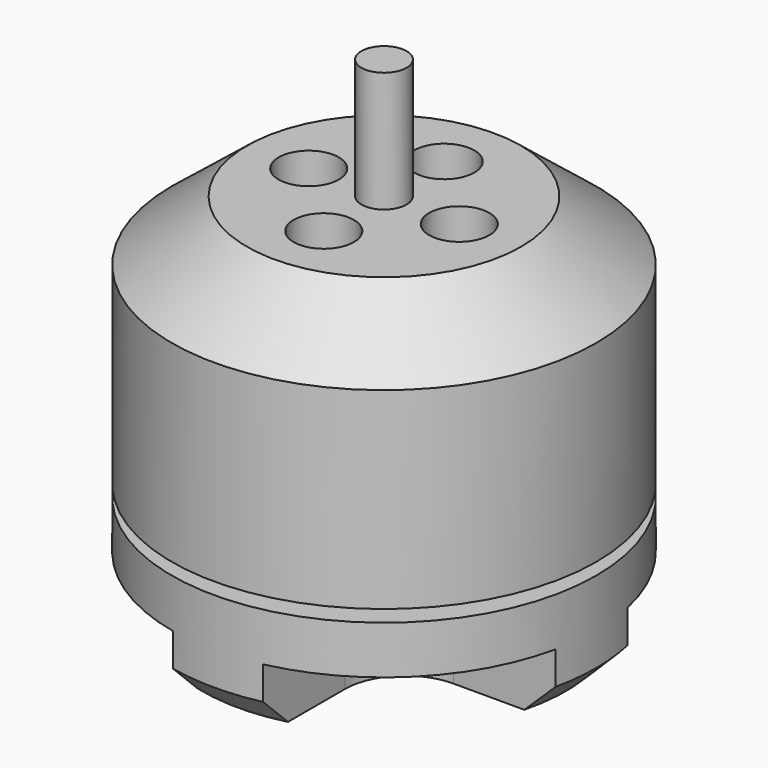
from build123d import *

# Parameters (mm, degrees)
F0_R      = 7.05
F0_R_2    = 4.5
F0_R_3    = 1
F0_R_4    = 0.75
F1_DEPTH  = 12.5
F2_SIZE2  = 2
F2_SIZE   = 2.5
F3_DEPTH  = 4
F4_DEPTH  = 5
F5_SIZE   = 1
F7_R      = 1
F8_DEPTH  = 2.5
F10_R     = 8.05
F11_DEPTH = 0.4


# Not quite as in the source:
# - a feature names something its author has since deleted; it is built from what else it names


with BuildPart() as f1:
    # F0 (on Top) → F1 (new body)
    with BuildSketch(Plane.XY):
        Circle(F0_R)
        Circle(F0_R_2, mode=Mode.SUBTRACT)
        Circle(F0_R_2)
        with Locations((0, -2.5)):
            Circle(F0_R_3, mode=Mode.SUBTRACT)
        with Locations((-2.5, 0)):
            Circle(F0_R_3, mode=Mode.SUBTRACT)
        Circle(F0_R_4, mode=Mode.SUBTRACT)
        with Locations((2.5, 0)):
            Circle(F0_R_3, mode=Mode.SUBTRACT)
        with Locations((0, 2.5)):
            Circle(F0_R_3, mode=Mode.SUBTRACT)
        with Locations((0, 2.5)):
            Circle(F0_R_3)
        with Locations((2.5, 0)):
            Circle(F0_R_3)
        with Locations((-2.5, 0)):
            Circle(F0_R_3)
        with Locations((0, -2.5)):
            Circle(F0_R_3)
        Circle(F0_R_4)
    extrude(amount=-F1_DEPTH)

    # F2
    f2_edges = [f1.edges().sort_by_distance(p)[0] for p in [
        (-7.05, 0, 0),
    ]]
    f2_side = f1.faces().sort_by_distance((0, 0, 0))[0]
    chamfer(f2_edges, length=F2_SIZE, length2=F2_SIZE2, reference=f2_side)

    # F0 (on Top) → F3 (join)
    with BuildSketch(Plane.XY):
        Circle(F0_R_4)
    extrude(amount=F3_DEPTH)

    # F0 (on Top) → F4 (cut)
    with BuildSketch(Plane.XY):
        with Locations((-2.5, 0)):
            Circle(F0_R_3)
        with Locations((2.5, 0)):
            Circle(F0_R_3)
        with Locations((0, 2.5)):
            Circle(F0_R_3)
        with Locations((0, -2.5)):
            Circle(F0_R_3)
    extrude(amount=-F4_DEPTH, mode=Mode.SUBTRACT)

    # F5
    f5_edges = [f1.edges().sort_by_distance(p)[0] for p in [
        (-7.05, 0, -12.5),
    ]]
    chamfer(f5_edges, length=F5_SIZE)

    # F7 (on offset) → F8 (cut)
    with BuildSketch(Plane(origin=(0, 0, -12.9), x_dir=(1, 0, 0), z_dir=(0, 0, -1))):
        with Locations((4.5, 0)):
            Circle(F7_R)
        with Locations((0, 4.5)):
            Circle(F7_R)
        with Locations((-4.5, 0)):
            Circle(F7_R)
        with Locations((0, -4.5)):
            Circle(F7_R)
        with BuildLine():
            Line((12.5710678119, -1.5), (3.5, -1.5))
            ThreePointArc((3.5, -1.5), (2.0857864376, -2.0857864376), (1.5, -3.5))
            Line((1.5, -3.5), (1.5, -12.5710678119))
            Line((1.5, -12.5710678119), (12.5710678119, -1.5))
        make_face()
        with BuildLine():
            Line((12.5710678119, 1.5), (1.5, 12.5710678119))
            Line((1.5, 12.5710678119), (1.5, 3.5))
            ThreePointArc((1.5, 3.5), (2.0857864376, 2.0857864376), (3.5, 1.5))
            Line((3.5, 1.5), (12.5710678119, 1.5))
        make_face()
        with BuildLine():
            Line((-1.5, 12.5710678119), (-12.5710678119, 1.5))
            Line((-12.5710678119, 1.5), (-3.5, 1.5))
            ThreePointArc((-3.5, 1.5), (-2.0857864376, 2.0857864376), (-1.5, 3.5))
            Line((-1.5, 3.5), (-1.5, 12.5710678119))
        make_face()
        with BuildLine():
            Line((-12.5710678119, -1.5), (-1.5, -12.5710678119))
            Line((-1.5, -12.5710678119), (-1.5, -3.5))
            ThreePointArc((-1.5, -3.5), (-2.0857864376, -2.0857864376), (-3.5, -1.5))
            Line((-3.5, -1.5), (-12.5710678119, -1.5))
        make_face()
    extrude(amount=-F8_DEPTH, mode=Mode.SUBTRACT)

    # F10 (on offset) → F11 (cut)
    with BuildSketch(Plane(origin=(0, 0, -8.8), x_dir=(1, 0, 0), z_dir=(0, 0, -1))):
        Circle(F10_R)
    extrude(amount=-F11_DEPTH, mode=Mode.SUBTRACT)


solid = f1.part
